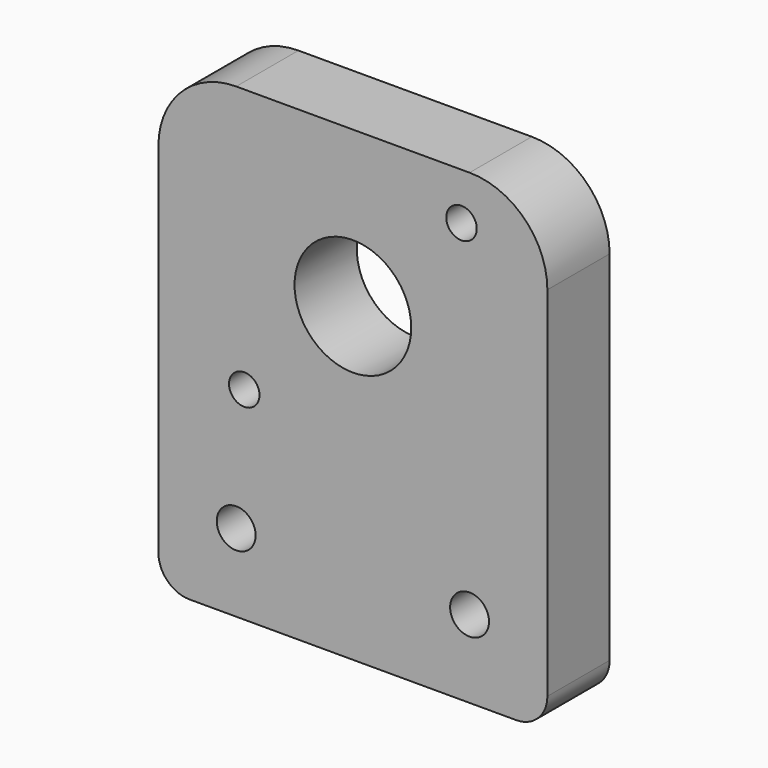
from build123d import *

# Parameters (mm, degrees)
F0_R     = 3.175
F0_R_2   = 2.4892
F0_R_3   = 9.525
F1_DEPTH = 12.7
F2_R     = 5.08


with BuildPart() as f1:
    # F0 (on Front) → F1 (new body)
    with BuildSketch(Plane.XZ):
        with BuildLine():
            Line((-31.75, -25.4), (31.75, -25.4))
            Line((31.75, -25.4), (31.75, 38.1))
            ThreePointArc((31.75, 38.1), (28.0302561211, 47.0802561211), (19.05, 50.8))
            Line((19.05, 50.8), (-19.05, 50.8))
            ThreePointArc((-19.05, 50.8), (-28.0302561211, 47.0802561211), (-31.75, 38.1))
            Line((-31.75, 38.1), (-31.75, -25.4))
        make_face()
        with Locations((-19.05, -12.7)):
            Circle(F0_R, mode=Mode.SUBTRACT)
        with Locations((-17.7292, 7.6708)):
            Circle(F0_R_2, mode=Mode.SUBTRACT)
        with Locations((19.05, -12.7)):
            Circle(F0_R, mode=Mode.SUBTRACT)
        with Locations((0, 25.4)):
            Circle(F0_R_3, mode=Mode.SUBTRACT)
        with Locations((17.7292, 43.1292)):
            Circle(F0_R_2, mode=Mode.SUBTRACT)
    extrude(amount=F1_DEPTH)

    # F2
    f2_edges = [f1.edges().sort_by_distance(p)[0] for p in [
        (31.75, -6.35, -25.4),
        (-31.75, -6.35, -25.4),
    ]]
    fillet(f2_edges, radius=F2_R)


solid = f1.part
